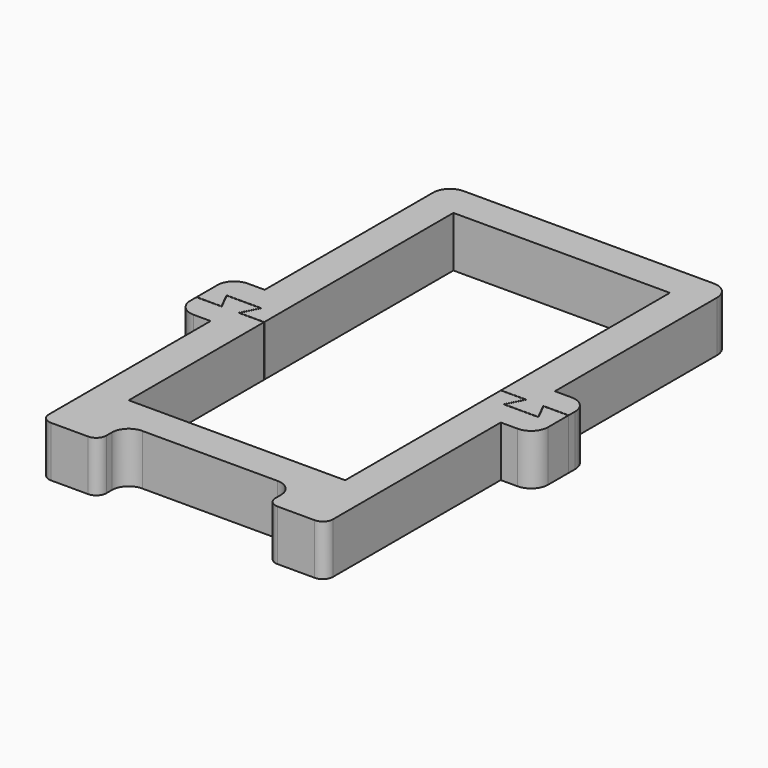
from build123d import *

# Parameters (mm, degrees)
F0_W          = 64
F0_H          = 120
F1_DEPTH      = 15
F2_R          = 3
F3_R          = 5
F4_W          = 20
F4_H          = 15
F5_DEPTH      = 10
F6_W          = 20
F6_H          = 15
F7_DEPTH      = 10
F9_DEPTH      = 15.001
F9_DEPTH_BACK = 191
F10_R         = 5


# Not quite as in the source:
# - an extrude ends at something that could not be found from the text; its depth is read off the source's solid


with BuildPart() as f1:
    # F0 (on Top) → F1 (new body)
    with BuildSketch(Plane.XY):
        Polygon((42, -75), (42, 75), (-42, 75), (-42, -75), (-25, -75), (-25, -65), (25, -65), (25, -75), align=None)
        with Locations((0, 5)):
            Rectangle(F0_W, F0_H, mode=Mode.SUBTRACT)
    extrude(amount=F1_DEPTH)

    # F2
    f2_edges = [f1.edges().sort_by_distance(p)[0] for p in [
        (25, -75, 7.5),
        (42, -75, 7.5),
        (-25, -75, 7.5),
        (-42, -75, 7.5),
    ]]
    fillet(f2_edges, radius=F2_R)

    # F3
    f3_edges = [f1.edges().sort_by_distance(p)[0] for p in [
        (-25, -65, 7.5),
        (25, -65, 7.5),
        (-42, 75, 7.5),
        (42, 75, 7.5),
    ]]
    fillet(f3_edges, radius=F3_R)

    # F4 (on face) → F5 (join)
    with BuildSketch(Plane(origin=(-42, 0, 0), x_dir=(0, -1, 0), z_dir=(-1, 0, 0))):
        with Locations((2.2429061755, 7.5)):
            Rectangle(F4_W, F4_H)
    extrude(amount=F5_DEPTH)

    # F6 (on face) → F7 (join)
    with BuildSketch(Plane.YZ.offset(42)):
        with Locations((0, 7.5)):
            Rectangle(F6_W, F6_H)
    extrude(amount=F7_DEPTH)

    # F8 (on face) → F9 (cut, two sides)
    with BuildSketch(Plane.XY.offset(15)) as f9_sk:
        Polygon((-44.5, -5), (-47, 0), (-37, 0), (-39.5, -5), (-31.7807010276, -5), (-31.188910827, -5), (-31.188910827, -4.9), (-39.3381966011, -4.9), (-36.8381966011, 0.1), (-47.1618033989, 0.1), (-44.6618033989, -4.9), (-53.2719284122, -4.9), (-53.2719284122, -5), align=None)
        Polygon((44.6618033989, 2.5), (52.811089173, 2.5), (52.811089173, 2.6), (44.5, 2.6), (47, -2.4), (37, -2.4), (39.5, 2.6), (30.7280715878, 2.6), (30.7280715878, 2.5), (39.3381966011, 2.5), (36.8381966011, -2.5), (47.1618033989, -2.5), align=None)
    extrude(amount=-F9_DEPTH, mode=Mode.SUBTRACT)
    extrude(f9_sk.sketch, amount=F9_DEPTH_BACK, mode=Mode.SUBTRACT)

    # F10
    f10_edges = [f1.edges().sort_by_distance(p)[0] for p in [
        (52, -10, 7.5),
        (52, 10, 7.5),
        (-52, 7.757094, 7.5),
        (-52, -12.242906, 7.5),
    ]]
    fillet(f10_edges, radius=F10_R)


solid = f1.part
